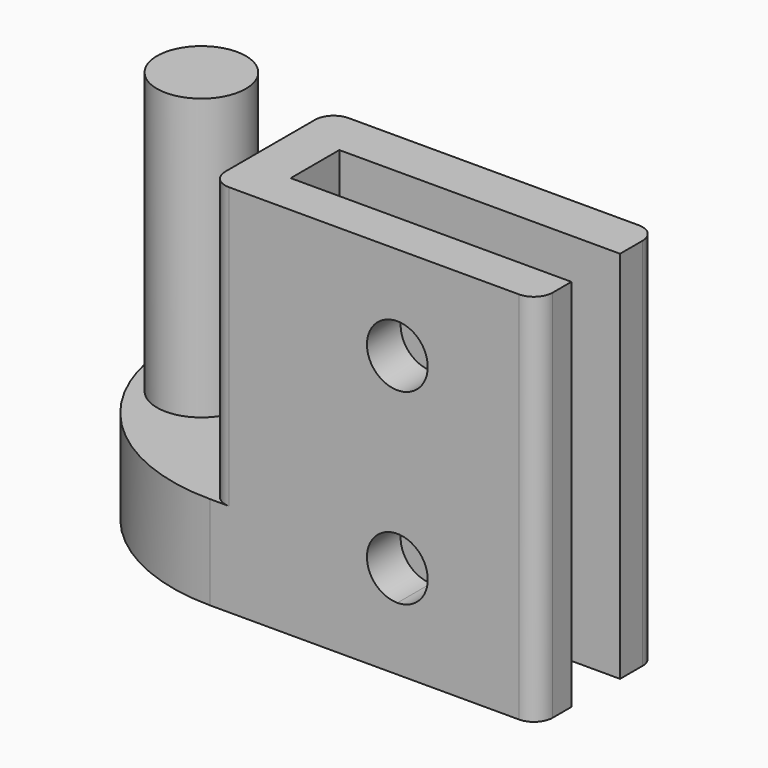
from build123d import *

# Parameters (mm, degrees)
F1_DEPTH = 20
F0_R     = 2.375
F2_DEPTH = 5
F3_DEPTH = 20
F4_R     = 1
F6_DEPTH = 8.5
F7_R     = 9.99999


# Not quite as in the source:
# - a fillet or chamfer is up to 0.001 mm smaller than in the source, because OpenCascade refuses the exact size


with BuildPart() as f1:
    # F0 (on Top) → F1 (new body)
    with BuildSketch(Plane.XY):
        Polygon((7.5, -3.875), (7.5, -1.625), (-7.5, -1.625), (-7.5, 1.625), (7.5, 1.625), (7.5, 4.125), (-10, 4.125), (-10, -3.875), align=None)
    extrude(amount=F1_DEPTH)

    # F0 (on Top) → F2 (join)
    with BuildSketch(Plane.XY):
        Polygon((-20, -3.875), (-10, -3.875), (-10, 4.125), (-13, 4.125), (-13, 7.125), (-20, 7.125), align=None)
        with Locations((-16.3791049272, 3.5122572444)):
            Circle(F0_R, mode=Mode.SUBTRACT)
    extrude(amount=F2_DEPTH)

    # F0 (on Top) → F3 (join)
    with BuildSketch(Plane.XY):
        with Locations((-16.3791049272, 3.5122572444)):
            Circle(F0_R)
    extrude(amount=F3_DEPTH)

    # F4
    f4_edges = [f1.edges().sort_by_distance(p)[0] for p in [
        (-20, 7.125, 2.5),
        (7.5, 4.125, 10),
        (7.5, -3.875, 10),
        (-10, 4.125, 12.5),
        (-10, -3.875, 12.5),
        (-13, 7.125, 2.5),
        (-13, 4.125, 2.5),
    ]]
    fillet(f4_edges, radius=F4_R)

    # F5 (on face) → F6 (cut)
    with BuildSketch(Plane.XZ.offset(3.875)):
        with BuildLine():
            ThreePointArc((1.625, 15), (1.1490485194, 16.1490485194), (0, 16.625))
            ThreePointArc((0, 16.625), (-1.1490485194, 13.8509514806), (1.625, 15))
        make_face()
        with BuildLine():
            ThreePointArc((1.625, 5), (-1.1490485194, 6.1490485194), (0, 3.375))
            ThreePointArc((0, 3.375), (1.1490485194, 3.8509514806), (1.625, 5))
        make_face()
    extrude(amount=-F6_DEPTH, mode=Mode.SUBTRACT)

    # F7 (radius 10 in the source; OpenCascade refuses exactly that, so slightly less here)
    f7_edges = [f1.edges().sort_by_distance(p)[0] for p in [
        (-20, -3.875, 2.5),
    ]]
    fillet(f7_edges, radius=F7_R)


solid = f1.part
